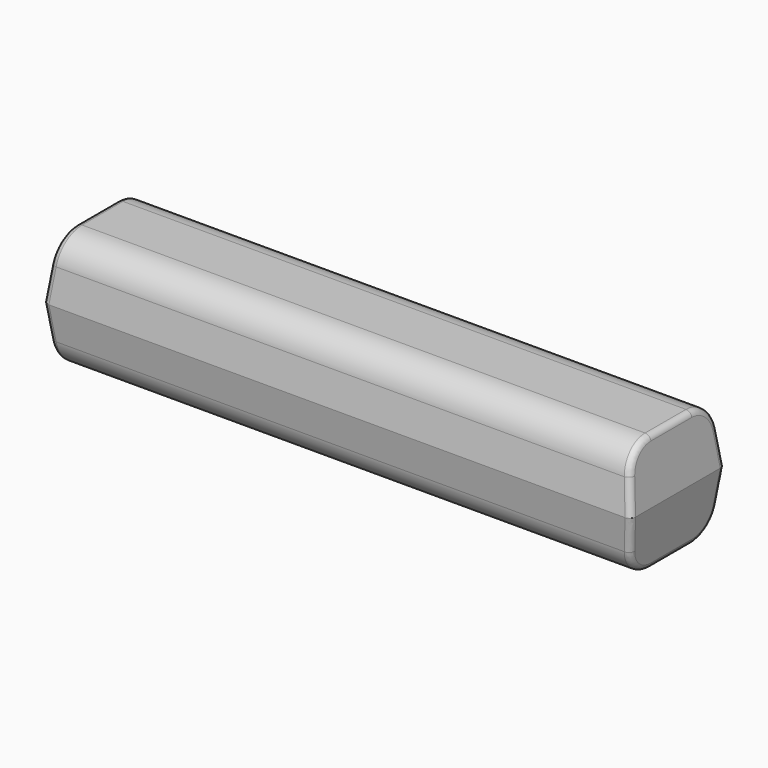
from build123d import *

# Parameters (mm, degrees)
F0_W     = 100
F0_H     = 20
F1_DEPTH = 10
F1_TAPER = 7
F2_R     = 5
F3_F1_R  = 1
F3_F2_R  = 1
F3_F3_R  = 0.9999
F3_F4_R  = 0.9999
F5_R     = 6
F6_DEPTH = 25


# Not quite as in the source:
# - two fillets or chamfers of one size are made in one step
# - a fillet or chamfer is up to 0.001 mm smaller than in the source, because OpenCascade refuses the exact size


with BuildPart() as f1:
    # F0 (on Top) → F1 (new body, symmetric)
    with BuildSketch(Plane.XY):
        with Locations((50, -10)):
            Rectangle(F0_W, F0_H)
    extrude(amount=F1_DEPTH, both=True, taper=F1_TAPER)

    # F2
    f2_edges = [f1.edges().sort_by_distance(p)[0] for p in [
        (50, -1.227846, -10),
        (50, -1.227846, 10),
        (50, -18.772154, -10),
        (50, -18.772154, 10),
    ]]
    fillet(f2_edges, radius=F2_R)

    # F3: fillet of radius 1 on 20 edges, made by hand

    # F3_f1
    f3_f1_edges = [f1.edges().sort_by_distance(p)[0] for p in [
        (0.3443705868, -0.3443705868, -2.8046733585),
        (0.3443705868, -19.6556294132, -2.8046733585),
        (1.0740434507, -17.6586834505, -8.7473819414),
        (1.227845609, -10, -10),
        (1.0740434507, -2.3413165503, -8.7473819411),
    ]]
    fillet(f3_f1_edges, radius=F3_F1_R)

    # F3_f2
    f3_f2_edges = [f1.edges().sort_by_distance(p)[0] for p in [
        (99.6556294132, -0.3443705868, -2.8046733585),
        (98.9259565281, -2.3413167447, -8.7473821136),
        (98.772154391, -10, -10),
        (99.6556294132, -19.6556294132, -2.8046733585),
        (98.9259565316, -17.6586832871, -8.7473820856),
    ]]
    fillet(f3_f2_edges, radius=F3_F2_R)

    # F3_f3 (radius 1 in the source; OpenCascade refuses exactly that, so slightly less here)
    f3_f3_edges = [f1.edges().sort_by_distance(p)[0] for p in [
        (99.5831739882, -0.4168260118, 3.3947754399),
        (99.5831739883, -19.5831739883, 3.3947754399),
        (98.9262761989, -17.6616283093, 8.7447786039),
        (98.772154391, -10, 10),
        (98.9262761989, -2.3383716907, 8.7447786039),
    ]]
    fillet(f3_f3_edges, radius=F3_F3_R)

    # F3_f4 (radius 1 in the source; OpenCascade refuses exactly that, so slightly less here)
    f3_f4_edges = [f1.edges().sort_by_distance(p)[0] for p in [
        (0.4168258896, -0.4168258896, 3.3947744453),
        (1.0737238011, -2.3383716907, 8.7447786039),
        (1.227845609, -10, 10),
        (0.4168260119, -19.5831739881, 3.3947754414),
        (1.0737238011, -17.6616283093, 8.7447786039),
    ]]
    fillet(f3_f4_edges, radius=F3_F4_R)

    # F5 (on Right) → F6 (cut)
    with BuildSketch(Plane.YZ):
        with Locations((-10, 0)):
            Circle(F5_R)
    extrude(amount=F6_DEPTH, mode=Mode.SUBTRACT)


solid = f1.part
